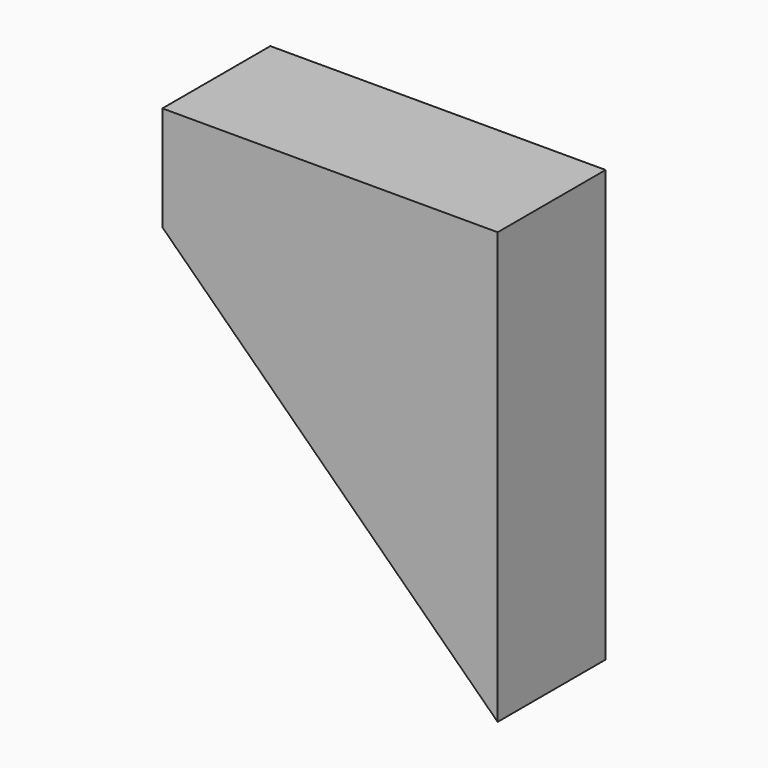
from build123d import *

# Parameters (mm, degrees)
F1_DEPTH = 25.4


# Not quite as in the source:
# - a feature of the source that left no trace in its solid (it failed there, or was rolled back) is left out


with BuildPart() as f1:
    # F0 (on Front) → F1 (new body)
    with BuildSketch(Plane.XZ):
        Polygon((-32.8028090298, 55.1706478), (-32.8028090298, 35.4637503624), (30.3142257035, -25.9798299521), (30.3142257035, 55.1706478), align=None)
    extrude(amount=F1_DEPTH)


solid = f1.part
